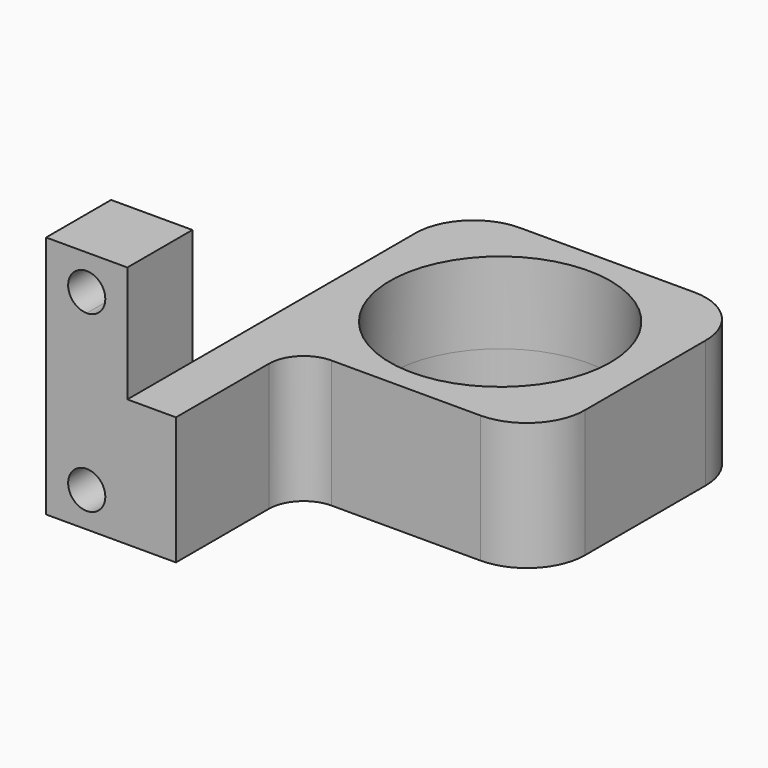
from build123d import *

# Parameters (mm, degrees)
F0_W     = 32
F0_H     = 36
F1_DEPTH = 4
F2_R     = 9.5
F2_W     = 7
F2_H     = 29
F2_W_2   = 20.817460835
F2_H_2   = 13
F3_DEPTH = 25
F4_W     = 7
F4_H     = 7
F4_R     = 9.5
F5_DEPTH = 7
F6_DEPTH = 17
F8_DEPTH = 25
F9_R     = 5
F10_R    = 3


# Not quite as in the source:
# - a feature of the source that left no trace in its solid (it failed there, or was rolled back) is left out


with BuildPart() as f1:
    # F0 (on Top) → F1 (new body)
    with BuildSketch(Plane.XY):
        with Locations((16, 18)):
            Rectangle(F0_W, F0_H)
    extrude(amount=F1_DEPTH)

    # F2 (on face) → F3 (cut)
    with BuildSketch(Plane.XY.offset(4)):
        with Locations((19.5, 24.5)):
            Circle(F2_R)
        with Locations((3.5, 21.5)):
            Rectangle(F2_W, F2_H)
        with Locations((21.5912695825, 6.5)):
            Rectangle(F2_W_2, F2_H_2)
    extrude(amount=-F3_DEPTH, mode=Mode.SUBTRACT)

    # F4 (on face) → F5 (join)
    with BuildSketch(Plane.XY.offset(4)):
        with Locations((3.5, 3.5)):
            Rectangle(F4_W, F4_H)
        Polygon((7, 36), (7, 7), (7, 0), (11.182539165, 0), (11.182539165, 13), (32, 13), (32, 36), align=None)
        with Locations((19.5, 24.5)):
            Circle(F4_R, mode=Mode.SUBTRACT)
    extrude(amount=F5_DEPTH)

    # F4 (on face) → F6 (join)
    with BuildSketch(Plane.XY.offset(4)):
        with Locations((3.5, 3.5)):
            Rectangle(F4_W, F4_H)
    extrude(amount=F6_DEPTH)

    # F7 (on face) → F8 (cut)
    with BuildSketch(Plane.XZ):
        with BuildLine():
            ThreePointArc((5.1, 3), (4.6313708499, 4.1313708499), (3.5, 4.6))
            ThreePointArc((3.5, 4.6), (2.3686291501, 1.8686291501), (5.1, 3))
        make_face()
        with BuildLine():
            ThreePointArc((5.1, 18), (2.3686291501, 19.1313708499), (3.5, 16.4))
            ThreePointArc((3.5, 16.4), (4.6313708499, 16.8686291501), (5.1, 18))
        make_face()
    extrude(amount=-F8_DEPTH, mode=Mode.SUBTRACT)

    # F9
    f9_edges = [f1.edges().sort_by_distance(p)[0] for p in [
        (32, 36, 5.5),
        (7, 36, 5.5),
        (32, 13, 5.5),
    ]]
    fillet(f9_edges, radius=F9_R)

    # F10
    f10_edges = [f1.edges().sort_by_distance(p)[0] for p in [
        (11.182539, 13, 5.5),
    ]]
    fillet(f10_edges, radius=F10_R)


solid = f1.part
